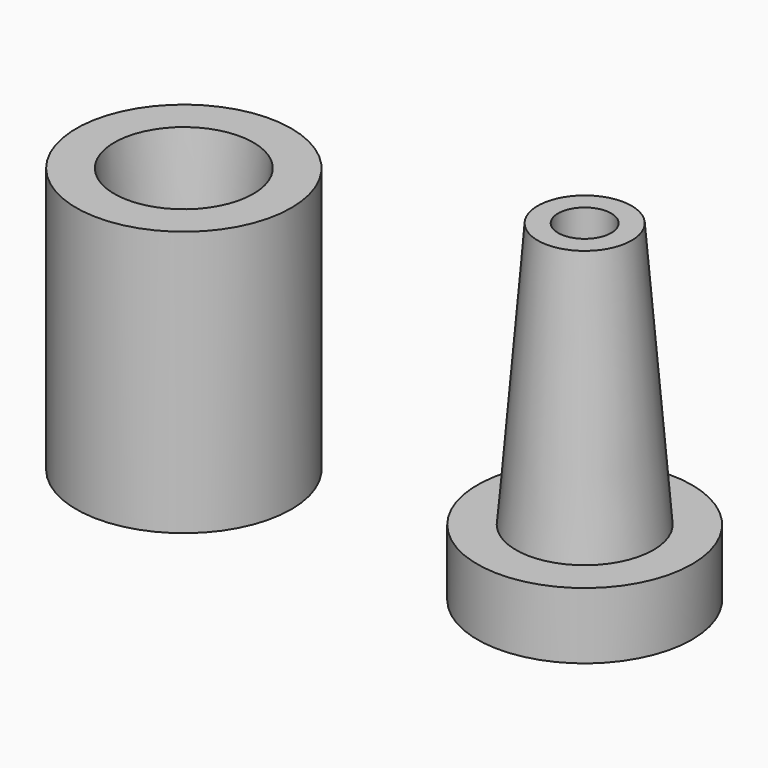
from build123d import *

# Parameters (mm, degrees)
F0_R          = 5.1470603346
F1_DEPTH      = 12.7
F2_R          = 3.3270987649
F3_DEPTH      = 12.7
F3_TAPER      = 5
F3_DEPTH_BACK = 25.4
F0_R_2        = 3.2884076422
F0_R_3        = 1.2711261933
F4_DEPTH      = 12.7
F5_SIZE2      = 12.69999
F5_SIZE       = 1.04139
F6_R          = 1.2647403263
F7_DEPTH      = 12.7
F0_R_4        = 5.137308395
F8_DEPTH      = 3.175


# Not quite as in the source:
# - a fillet or chamfer is up to 0.001 mm smaller than in the source, because OpenCascade refuses the exact size


with BuildPart() as f1:
    # F0 (on Top) → F1 (new body)
    with BuildSketch(Plane.XY):
        with Locations((-13.5284401476, 3.1272724736)):
            Circle(F0_R)
    extrude(amount=F1_DEPTH)

    # F2 (on face) → F3 (cut, two sides)
    with BuildSketch(Plane.XY.offset(12.7)) as f3_sk:
        with Locations((-13.5284401476, 3.1272724736)):
            Circle(F2_R)
    extrude(amount=-F3_DEPTH, taper=F3_TAPER, mode=Mode.SUBTRACT)
    extrude(f3_sk.sketch, amount=F3_DEPTH_BACK, mode=Mode.SUBTRACT)

    # F6 (on face) → F7 (cut)
    with BuildSketch(Plane.XY.offset(12.7)):
        with Locations((4.7591873445, 4.2478842661)):
            Circle(F6_R)
    extrude(amount=-F7_DEPTH, mode=Mode.SUBTRACT)


with BuildPart() as f4:
    # F0 (on Top) → F4 (new body)
    with BuildSketch(Plane.XY):
        with Locations((4.7591873445, 4.2478842661)):
            Circle(F0_R_2)
        with Locations((4.7591873445, 4.2478842661)):
            Circle(F0_R_3, mode=Mode.SUBTRACT)
    extrude(amount=F4_DEPTH)

    # F5 (size 1.0414 and 12.7 in the source; OpenCascade refuses exactly that, so slightly less here)
    f5_edges = [f4.edges().sort_by_distance(p)[0] for p in [
        (1.47078, 4.247884, 12.7),
    ]]
    f5_side = f4.faces().sort_by_distance((1.56379, 4.247884, 12.7))[0]
    chamfer(f5_edges, length=F5_SIZE, length2=F5_SIZE2, reference=f5_side)

    # F0 (on Top) → F8 (join)
    with BuildSketch(Plane.XY):
        with Locations((4.7591873445, 4.2478842661)):
            Circle(F0_R_4)
        with Locations((4.7591873445, 4.2478842661)):
            Circle(F0_R_2, mode=Mode.SUBTRACT)
        with Locations((4.7591873445, 4.2478842661)):
            Circle(F0_R_2)
        with Locations((4.7591873445, 4.2478842661)):
            Circle(F0_R_3, mode=Mode.SUBTRACT)
    extrude(amount=-F8_DEPTH)


with BuildPart() as f4_1:
    # F9: moved
    add(f4.part.moved(Location((0, 0, 3.175))))


solid = Compound([f1.part, f4_1.part])
